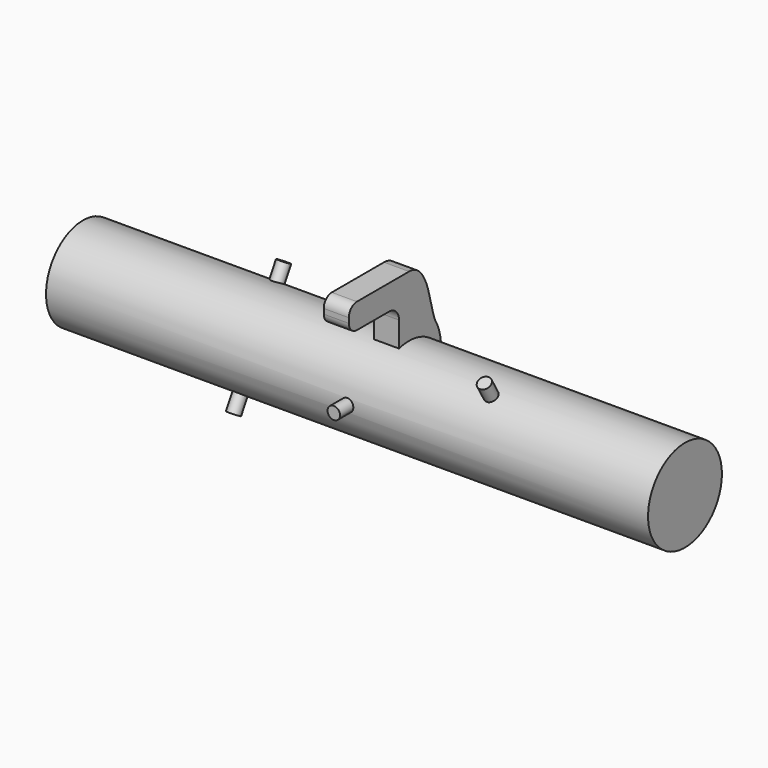
from build123d import *

# Parameters (mm, degrees)
F1_R      = 23.368
F4_DEPTH  = 152.4
F5_R      = 3.175
F8_DEPTH  = 25.4
F7_R      = 3.175
F9_DEPTH  = 25.4
F6_R      = 3.175
F10_DEPTH = 25.4
F11_DEPTH = 31.75
F12_DEPTH = 31.75
F13_DEPTH = 31.75
F15_DEPTH = 12.7
F16_R     = 5.08


# Not quite as in the source:
# - a variable given as a bare number and used for a length is read in inches; the dataset says mm whatever the document's units were


with BuildPart() as f4:
    # F1 (on Right) → F4 (new body, symmetric)
    with BuildSketch(Plane.YZ):
        Circle(F1_R)
    extrude(amount=F4_DEPTH, both=True)

    # F5 (on Front) → F8 (cut, symmetric)
    with BuildSketch(Plane.XZ):
        Circle(F5_R)
    extrude(amount=F8_DEPTH, both=True, mode=Mode.SUBTRACT)

    # F7 (on face) → F9 (cut, symmetric)
    with BuildSketch(Plane(origin=(0, 0, 0), x_dir=(1, 0, 0), z_dir=(0, -0.5, 0.8660254038))):
        with Locations((63.5, 0)):
            Circle(F7_R)
    extrude(amount=F9_DEPTH, both=True, mode=Mode.SUBTRACT)

    # F6 (on face) → F10 (cut, symmetric)
    with BuildSketch(Plane(origin=(0, 0, 0), x_dir=(1, 0, 0), z_dir=(0, 0.5, 0.8660254038))):
        with Locations((-63.5, 0)):
            Circle(F6_R)
    extrude(amount=F10_DEPTH, both=True, mode=Mode.SUBTRACT)


with BuildPart() as f11:
    # F6 (on face) → F11 (new body, symmetric)
    with BuildSketch(Plane(origin=(0, 0, 0), x_dir=(1, 0, 0), z_dir=(0, 0.5, 0.8660254038))):
        with Locations((-63.5, 0)):
            Circle(F6_R)
    extrude(amount=F11_DEPTH, both=True)


with BuildPart() as f12:
    # F5 (on Front) → F12 (new body, symmetric)
    with BuildSketch(Plane.XZ):
        Circle(F5_R)
    extrude(amount=F12_DEPTH, both=True)


with BuildPart() as f13:
    # F7 (on face) → F13 (new body, symmetric)
    with BuildSketch(Plane(origin=(0, 0, 0), x_dir=(1, 0, 0), z_dir=(0, -0.5, 0.8660254038))):
        with Locations((63.5, 0)):
            Circle(F7_R)
    extrude(amount=F13_DEPTH, both=True)


with BuildPart() as f15:
    # F14 (on Right) → F15 (new body)
    with BuildSketch(Plane.YZ):
        with BuildLine():
            Line((-6.35, 35.1886843546), (-6.35, 22.4886843546))
            ThreePointArc((-6.35, 22.4886843546), (0, 23.368), (6.35, 22.4886843546))
            Line((6.35, 22.4886843546), (6.35, 35.1886843546))
            ThreePointArc((6.35, 35.1886843546), (12.2295840817, 31.0651383233), (16.7200072547, 25.460743568))
            add(Edge.make_bspline(
                [(0, 54.2386843546), (12.7, 54.2386843546), (13.4898950697, 30.9278154783), (16.7200072547, 25.460743568)],
                knots=[0, 0, 0, 0, 33.2825557689, 33.2825557689, 33.2825557689, 33.2825557689], degree=3))
            Line((0, 54.2386843546), (-38.1, 54.2386843546))
            Line((-38.1, 54.2386843546), (-38.1, 41.5386843546))
            Line((-38.1, 41.5386843546), (-12.7, 41.5386843546))
            ThreePointArc((-12.7, 41.5386843546), (-8.2098719395, 39.6788124151), (-6.35, 35.1886843546))
        make_face()
        with BuildLine():
            ThreePointArc((6.35, 22.4886843546), (14.3494315983, 18.4433521033), (20.2372816356, 11.684))
            ThreePointArc((20.2372816356, 11.684), (19.4623116998, 18.823507157), (16.7200072547, 25.460743568))
            ThreePointArc((16.7200072547, 25.460743568), (12.2295840817, 31.0651383233), (6.35, 35.1886843546))
            Line((6.35, 35.1886843546), (6.35, 22.4886843546))
        make_face()
    extrude(amount=F15_DEPTH)

    # F16
    f16_edges = [f15.edges().sort_by_distance(p)[0] for p in [
        (6.35, -38.1, 54.238684),
        (6.35, -38.1, 41.538684),
    ]]
    fillet(f16_edges, radius=F16_R)


solid = Compound([f4.part, f11.part, f12.part, f13.part, f15.part])
